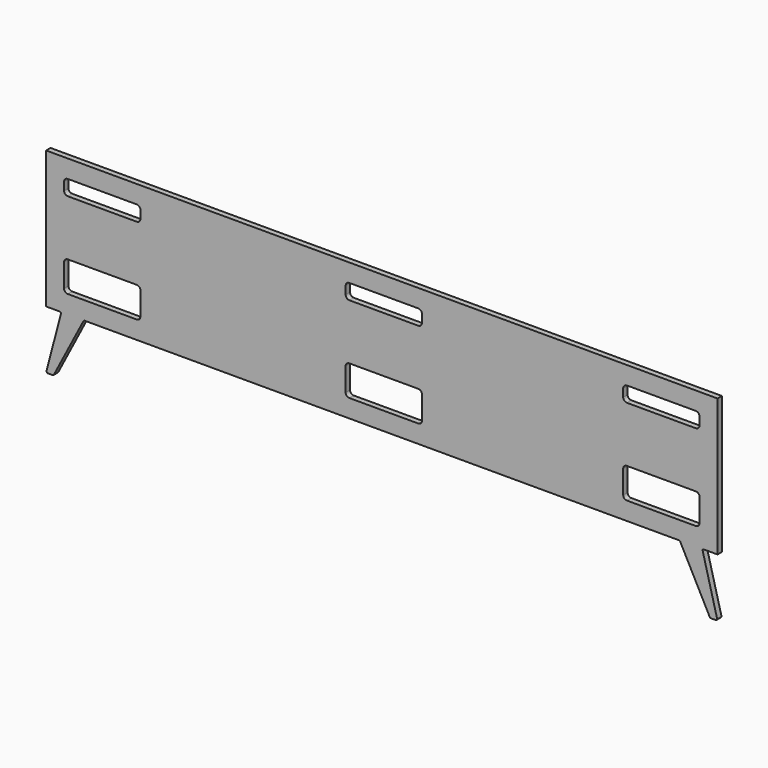
from build123d import *

# Parameters (mm, degrees)
F0_W     = 9
F0_H     = 432
F0_H_2   = 9
F1_DEPTH = 18


# Not quite as in the source:
# - a feature names something its author has since deleted; it is built from what else it names


with BuildPart() as f1:
    # F0 (on Front) → F1 (new body)
    with BuildSketch(Plane.XZ):
        Polygon((0, 75.8756743552), (-1100, 75.8756743552), (-1100, 66.8756743552), (-1091, 66.8756743552), (0, 66.8756743552), (1091, 66.8756743552), (1091, 75.8756743552), align=None)
        with BuildLine():
            Line((-973.3476458471, -374.1243256448), (-1054.6076226562, -374.1243256448))
            ThreePointArc((-1054.6076226562, -374.1243256448), (-1051.7483407187, -375.721921149), (-1051.265639742, -378.9614896944))
            Line((-1051.265639742, -378.9614896944), (-1098.3606008427, -558.954299013))
            ThreePointArc((-1098.3606008427, -558.954299013), (-1097.4812264988, -563.2754093644), (-1093.523436793, -565.219938755))
            Line((-1093.523436793, -565.219938755), (-1078.8076104242, -565.219938755))
            ThreePointArc((-1078.8076104242, -565.219938755), (-1076.2129629213, -564.4940239596), (-1074.371712623, -562.5270604893))
            Line((-1074.371712623, -562.5270604893), (-977.7835436484, -376.8172039105))
            ThreePointArc((-977.7835436484, -376.8172039105), (-975.94229335, -374.8502404402), (-973.3476458471, -374.1243256448))
        make_face()
        with BuildLine():
            Line((1100, 66.8756743552), (1091, 66.8756743552))
            Line((1091, 66.8756743552), (1091, -365.0378882885))
            Line((1091, -365.0378882885), (1091, -365.1243256448))
            Line((1091, -365.1243256448), (0, -365.1243256448))
            Line((0, -365.1243256448), (-1091, -365.1243256448))
            Line((-1091, -365.1243256448), (-1091, -374.1243256448))
            Line((-1091, -374.1243256448), (-1055, -374.1243256448))
            ThreePointArc((-1055, -374.1243256448), (-1054.8038113281, -374.1191399972), (-1054.6076226562, -374.1243256448))
            Line((-1054.6076226562, -374.1243256448), (-973.3476458471, -374.1243256448))
            Line((-973.3476458471, -374.1243256448), (0, -374.1243256448))
            Line((0, -374.1243256448), (973.3476458471, -374.1243256448))
            Line((973.3476458471, -374.1243256448), (1054.6076226562, -374.1243256448))
            ThreePointArc((1054.6076226562, -374.1243256448), (1054.8038113281, -374.1191399972), (1055, -374.1243256448))
            Line((1055, -374.1243256448), (1100, -374.1243256448))
            Line((1100, -374.1243256448), (1100, 66.8756743552))
        make_face()
        with Locations((-1095.5, -149.1243256448)):
            Rectangle(F0_W, F0_H)
        with Locations((-1095.5, -369.6243256448)):
            Rectangle(F0_W, F0_H_2)
        with Locations((1095.5, 71.3756743552)):
            Rectangle(F0_W, F0_H_2)
        with BuildLine():
            ThreePointArc((1051.265639742, -378.9614896944), (1051.7483407187, -375.721921149), (1054.6076226562, -374.1243256448))
            Line((1054.6076226562, -374.1243256448), (973.3476458471, -374.1243256448))
            ThreePointArc((973.3476458471, -374.1243256448), (975.94229335, -374.8502404402), (977.7835436484, -376.8172039105))
            Line((977.7835436484, -376.8172039105), (1074.371712623, -562.5270604893))
            ThreePointArc((1074.371712623, -562.5270604893), (1076.2129629213, -564.4940239596), (1078.8076104242, -565.219938755))
            Line((1078.8076104242, -565.219938755), (1093.523436793, -565.219938755))
            ThreePointArc((1093.523436793, -565.219938755), (1097.4812264988, -563.2754093644), (1098.3606008427, -558.954299013))
            Line((1098.3606008427, -558.954299013), (1051.265639742, -378.9614896944))
        make_face()
        Polygon((0, 66.8756743552), (-1091, 66.8756743552), (-1091, -365.1243256448), (0, -365.1243256448), (1091, -365.1243256448), (1091, -365.0378882885), (1091, 66.8756743552), align=None)
        with BuildLine():
            ThreePointArc((-1041, -227.1243239641), (-1037.4852813742, -218.6390425899), (-1029, -215.1243239641))
            Line((-1029, -215.1243239641), (-803, -215.1243239641))
            ThreePointArc((-803, -215.1243239641), (-794.5147186258, -218.6390425899), (-791, -227.1243239641))
            Line((-791, -227.1243239641), (-791, -303.1243256448))
            ThreePointArc((-791, -303.1243256448), (-794.5147186258, -311.609607019), (-803, -315.1243256448))
            Line((-803, -315.1243256448), (-1029, -315.1243256448))
            ThreePointArc((-1029, -315.1243256448), (-1037.4852813742, -311.609607019), (-1041, -303.1243256448))
            Line((-1041, -303.1243256448), (-1041, -227.1243239641))
        make_face(mode=Mode.SUBTRACT)
        with BuildLine():
            ThreePointArc((-118.4479668736, -227.1243239641), (-114.9332482479, -218.6390425899), (-106.4479668736, -215.1243239641))
            Line((-106.4479668736, -215.1243239641), (119.5520331264, -215.1243239641))
            ThreePointArc((119.5520331264, -215.1243239641), (128.0373145006, -218.6390425899), (131.5520331264, -227.1243239641))
            Line((131.5520331264, -227.1243239641), (131.5520331264, -303.1243256448))
            ThreePointArc((131.5520331264, -303.1243256448), (128.0373145006, -311.609607019), (119.5520331264, -315.1243256448))
            Line((119.5520331264, -315.1243256448), (-106.4479668736, -315.1243256448))
            ThreePointArc((-106.4479668736, -315.1243256448), (-114.9332482479, -311.609607019), (-118.4479668736, -303.1243256448))
            Line((-118.4479668736, -303.1243256448), (-118.4479668736, -227.1243239641))
        make_face(mode=Mode.SUBTRACT)
        with BuildLine():
            Line((791, -303.1243256448), (791, -227.1243239641))
            ThreePointArc((791, -227.1243239641), (794.5147186258, -218.6390425899), (803, -215.1243239641))
            Line((803, -215.1243239641), (1029, -215.1243239641))
            ThreePointArc((1029, -215.1243239641), (1037.4852813742, -218.6390425899), (1041, -227.1243239641))
            Line((1041, -227.1243239641), (1041, -303.1243256448))
            ThreePointArc((1041, -303.1243256448), (1037.4852813742, -311.609607019), (1029, -315.1243256448))
            Line((1029, -315.1243256448), (803, -315.1243256448))
            ThreePointArc((803, -315.1243256448), (794.5147186258, -311.609607019), (791, -303.1243256448))
        make_face(mode=Mode.SUBTRACT)
        with BuildLine():
            ThreePointArc((-1041, 4.8756749481), (-1037.4852813742, 13.3609563223), (-1029, 16.8756749481))
            Line((-1029, 16.8756749481), (-803, 16.8756749481))
            ThreePointArc((-803, 16.8756749481), (-794.5147186258, 13.3609563223), (-791, 4.8756749481))
            Line((-791, 4.8756749481), (-791, -21.1243239343))
            ThreePointArc((-791, -21.1243239343), (-794.5147186258, -29.6096053086), (-803, -33.1243239343))
            Line((-803, -33.1243239343), (-1029, -33.1243239343))
            ThreePointArc((-1029, -33.1243239343), (-1037.4852813742, -29.6096053086), (-1041, -21.1243239343))
            Line((-1041, -21.1243239343), (-1041, 4.8756749481))
        make_face(mode=Mode.SUBTRACT)
        with BuildLine():
            ThreePointArc((-118.4479668736, 4.8756749481), (-114.9332482479, 13.3609563223), (-106.4479668736, 16.8756749481))
            Line((-106.4479668736, 16.8756749481), (119.5520331264, 16.8756749481))
            ThreePointArc((119.5520331264, 16.8756749481), (128.0373145006, 13.3609563223), (131.5520331264, 4.8756749481))
            Line((131.5520331264, 4.8756749481), (131.5520331264, -21.1243239343))
            ThreePointArc((131.5520331264, -21.1243239343), (128.0373145006, -29.6096053086), (119.5520331264, -33.1243239343))
            Line((119.5520331264, -33.1243239343), (-106.4479668736, -33.1243239343))
            ThreePointArc((-106.4479668736, -33.1243239343), (-114.9332482479, -29.6096053086), (-118.4479668736, -21.1243239343))
            Line((-118.4479668736, -21.1243239343), (-118.4479668736, 4.8756749481))
        make_face(mode=Mode.SUBTRACT)
        with BuildLine():
            Line((803, 16.8756749481), (1029, 16.8756749481))
            ThreePointArc((1029, 16.8756749481), (1037.4852813742, 13.3609563223), (1041, 4.8756749481))
            Line((1041, 4.8756749481), (1041, -21.1243239343))
            ThreePointArc((1041, -21.1243239343), (1037.4852813742, -29.6096053086), (1029, -33.1243239343))
            Line((1029, -33.1243239343), (803, -33.1243239343))
            ThreePointArc((803, -33.1243239343), (794.5147186258, -29.6096053086), (791, -21.1243239343))
            Line((791, -21.1243239343), (791, 4.8756749481))
            ThreePointArc((791, 4.8756749481), (794.5147186258, 13.3609563223), (803, 16.8756749481))
        make_face(mode=Mode.SUBTRACT)
    extrude(amount=F1_DEPTH)


solid = f1.part
